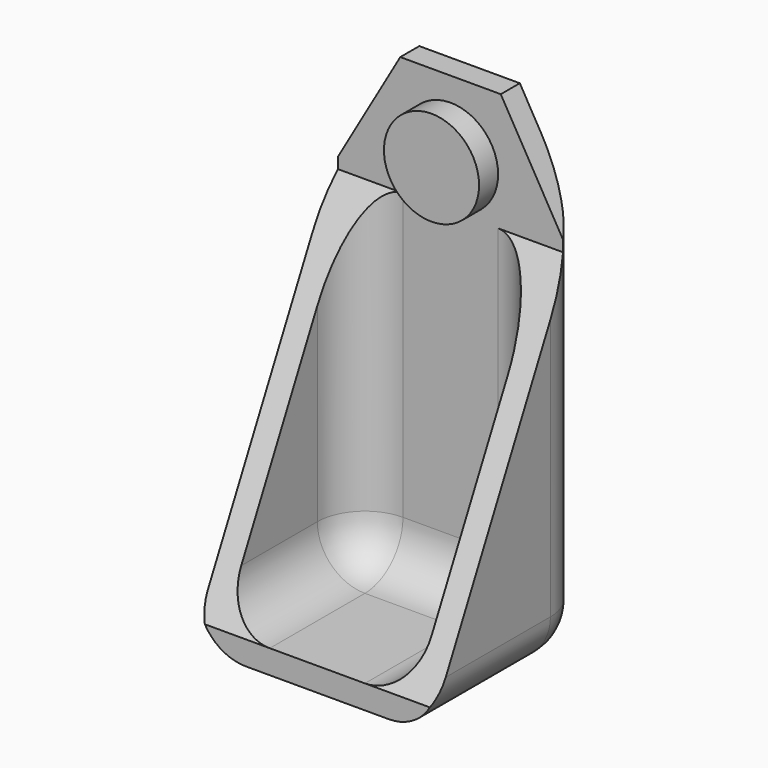
from build123d import *

# Parameters (mm, degrees)
F0_W          = 10
F0_H          = 15
F1_DEPTH      = 8
F2_W          = 8
F2_H          = 14
F3_DEPTH      = 14
F5_DEPTH      = 25
F7_DEPTH      = 1
F8_R          = 2
F9_DEPTH      = 1
F10_T1_DEPTH  = 4
F10_S5_W      = 2.04
F10_S5_H      = 2.04
F10_T6_DEPTH  = 2.04
F10_S11_W     = 2.04
F10_S11_H     = 2.04
F10_T12_DEPTH = 2.04
F10_T18_DEPTH = 10
F10_T23_DEPTH = 10
F10_T28_DEPTH = 17
F10_T33_DEPTH = 17
F10_T35_DEPTH = 6
F10_T37_DEPTH = 18
F10_T39_DEPTH = 11
F10_S43_W     = 2.04
F10_S43_H     = 2.04
F10_T44_DEPTH = 2.04
F10_S49_W     = 2.04
F10_S49_H     = 2.04
F10_T50_DEPTH = 2.04


# Not quite as in the source:
# - a fillet or chamfer that OpenCascade refuses, or shapes differently, is made with other operations: its cross-section is extruded or revolved along the edge and cut away or added


with BuildPart() as f1:
    # F0 (on Front) → F1 (new body)
    with BuildSketch(Plane.XZ):
        with Locations((0, 7.5)):
            Rectangle(F0_W, F0_H)
    extrude(amount=F1_DEPTH)

    # F2 (on face) → F3 (cut)
    with BuildSketch(Plane.XZ.offset(8)):
        with Locations((0, 8)):
            Rectangle(F2_W, F2_H)
    extrude(amount=-F3_DEPTH, mode=Mode.SUBTRACT)

    # F4 (on face) → F5 (cut)
    with BuildSketch(Plane(origin=(-5, 0, 0), x_dir=(0, -1, 0), z_dir=(-1, 0, 0))):
        Polygon((8, 15), (1, 15), (8, 1), align=None)
    extrude(amount=-F5_DEPTH, mode=Mode.SUBTRACT)

    # F6 (on face) → F7 (join)
    with BuildSketch(Plane(origin=(0, 0, 0), x_dir=(-1, 0, 0), z_dir=(0, 1, 0))):
        Polygon((4, 15), (5, 15), (2.1132486541, 20), (-2.1132486541, 20), (-5, 15), (-4, 15), (-4, 1), (4, 1), align=None)
    extrude(amount=-F7_DEPTH)

    # F8 (on face) → F9 (join)
    with BuildSketch(Plane.XZ.offset(1)):
        with Locations((0, 17)):
            Circle(F8_R)
    extrude(amount=F9_DEPTH)

    # F10: fillet of radius 2 on 12 edges, made by hand

    # F10_s2 → F10_t1 (join)
    with BuildSketch(Plane.YZ.offset(-2)):
        with BuildLine():
            ThreePointArc((-3, 1), (-1.5857864376, 1.5857864376), (-1, 3))
            Line((-1, 3), (-1, 1))
            Line((-1, 1), (-3, 1))
        make_face()
    extrude(amount=F10_T1_DEPTH)


with BuildPart() as f10_tool4:
    # F10_s5 → F10_t6 (new body)
    with BuildSketch(Plane.XY.offset(3)):
        with Locations((-3.02, -1.98)):
            Rectangle(F10_S5_W, F10_S5_H)
    extrude(amount=-F10_T6_DEPTH)

    # F10_s7 → F10_t8 (revolve, cut)
    with BuildSketch(Plane(origin=(-2, -3, 3), x_dir=(0.7071067812, -0.7071067812, 0), z_dir=(0.7071067812, 0.7071067812, 0))):
        with BuildLine():
            ThreePointArc((0, -2), (2, 0), (0, 2))
            Line((0, 2), (0, -2))
        make_face()
    revolve(axis=Axis((-2, -3, 3), (0, 0, -1)), mode=Mode.SUBTRACT)


with BuildPart() as f1_1:
    add(f1.part)

    # F10_t3: union F10_tool4
    add(f10_tool4.part)


with BuildPart() as f10_tool10:
    # F10_s11 → F10_t12 (new body)
    with BuildSketch(Plane.XY.offset(3)):
        with Locations((3.02, -1.98)):
            Rectangle(F10_S11_W, F10_S11_H)
    extrude(amount=-F10_T12_DEPTH)

    # F10_s13 → F10_t14 (revolve, cut)
    with BuildSketch(Plane(origin=(2, -3, 3), x_dir=(-0.7071067812, -0.7071067812, 0), z_dir=(0.7071067812, -0.7071067812, 0))):
        with BuildLine():
            ThreePointArc((0, -2), (2, 0), (0, 2))
            Line((0, 2), (0, -2))
        make_face()
    revolve(axis=Axis((2, -3, 3), (0, 0, -1)), mode=Mode.SUBTRACT)


with BuildPart() as f1_2:
    add(f1_1.part)

    # F10_t9: union F10_tool10
    add(f10_tool10.part)


with BuildPart() as f10_tool16:
    # F10_s17 → F10_t18 (new body)
    with BuildSketch(Plane.XZ.offset(13)):
        with BuildLine():
            ThreePointArc((-2, 1), (-3.4142135624, 1.5857864376), (-4, 3))
            Line((-4, 3), (-4, 1))
            Line((-4, 1), (-2, 1))
        make_face()
    extrude(amount=-F10_T18_DEPTH)

    split(bisect_by=Plane(origin=(0, -6.8, 3.4), x_dir=(1, 0, 0), z_dir=(0, 0.894427191, -0.4472135955)), keep=Keep.TOP)


with BuildPart() as f1_3:
    add(f1_2.part)

    # F10_t15: union F10_tool16
    add(f10_tool16.part)


with BuildPart() as f10_tool21:
    # F10_s22 → F10_t23 (new body)
    with BuildSketch(Plane.XZ.offset(13)):
        with BuildLine():
            ThreePointArc((2, 1), (3.4142135624, 1.5857864376), (4, 3))
            Line((4, 3), (4, 1))
            Line((4, 1), (2, 1))
        make_face()
    extrude(amount=-F10_T23_DEPTH)

    split(bisect_by=Plane(origin=(0, -6.8, 3.4), x_dir=(1, 0, 0), z_dir=(0, 0.894427191, -0.4472135955)), keep=Keep.TOP)


with BuildPart() as f1_4:
    add(f1_3.part)

    # F10_t20: union F10_tool21
    add(f10_tool21.part)


with BuildPart() as f10_tool26:
    # F10_s27 → F10_t28 (new body)
    with BuildSketch(Plane.XY.offset(20)):
        with BuildLine():
            ThreePointArc((2, -1), (3.4142135624, -1.5857864376), (4, -3))
            Line((4, -3), (4, -1))
            Line((4, -1), (2, -1))
        make_face()
    extrude(amount=-F10_T28_DEPTH)

    split(bisect_by=Plane(origin=(0, -6.8, 3.4), x_dir=(1, 0, 0), z_dir=(0, 0.894427191, -0.4472135955)), keep=Keep.TOP)


with BuildPart() as f1_5:
    add(f1_4.part)

    # F10_t25: union F10_tool26
    add(f10_tool26.part)


with BuildPart() as f10_tool31:
    # F10_s32 → F10_t33 (new body)
    with BuildSketch(Plane.XY.offset(3)):
        with BuildLine():
            ThreePointArc((-4, -3), (-3.4142135624, -1.5857864376), (-2, -1))
            Line((-2, -1), (-4, -1))
            Line((-4, -1), (-4, -3))
        make_face()
    extrude(amount=F10_T33_DEPTH)

    split(bisect_by=Plane(origin=(0, -6.8, 3.4), x_dir=(1, 0, 0), z_dir=(0, 0.894427191, -0.4472135955)), keep=Keep.TOP)


with BuildPart() as f1_6:
    add(f1_5.part)

    # F10_t30: union F10_tool31
    add(f10_tool31.part)

    # F10_s36 → F10_t35 (cut)
    with BuildSketch(Plane.YZ.offset(-3)):
        with BuildLine():
            ThreePointArc((-2, 0), (-0.5857864376, 0.5857864376), (0, 2))
            Line((0, 2), (0, 0))
            Line((0, 0), (-2, 0))
        make_face()
    extrude(amount=F10_T35_DEPTH, mode=Mode.SUBTRACT)

    # F10_s38 → F10_t37 (cut)
    with BuildSketch(Plane.XY.offset(2)):
        with BuildLine():
            ThreePointArc((-5, -2), (-4.4142135624, -0.5857864376), (-3, 0))
            Line((-3, 0), (-5, 0))
            Line((-5, 0), (-5, -2))
        make_face()
        with BuildLine():
            ThreePointArc((5, -2), (4.4142135624, -0.5857864376), (3, 0))
            Line((3, 0), (5, 0))
            Line((5, 0), (5, -2))
        make_face()
    extrude(amount=F10_T37_DEPTH, mode=Mode.SUBTRACT)

    # F10_s40 → F10_t39 (cut)
    with BuildSketch(Plane.XZ.offset(2)):
        with BuildLine():
            ThreePointArc((-5, 2), (-4.4142135624, 0.5857864376), (-3, 0))
            Line((-3, 0), (-5, 0))
            Line((-5, 0), (-5, 2))
        make_face()
        with BuildLine():
            ThreePointArc((5, 2), (4.4142135624, 0.5857864376), (3, 0))
            Line((3, 0), (5, 0))
            Line((5, 0), (5, 2))
        make_face()
    extrude(amount=F10_T39_DEPTH, mode=Mode.SUBTRACT)


with BuildPart() as f10_tool42:
    # F10_s43 → F10_t44 (new body)
    with BuildSketch(Plane.YZ.offset(-3)):
        with Locations((-0.98, 0.98)):
            Rectangle(F10_S43_W, F10_S43_H)
    extrude(amount=-F10_T44_DEPTH)

    # F10_s45 → F10_t46 (revolve, cut)
    with BuildSketch(Plane(origin=(-3, -2, 2), x_dir=(0, -0.7071067812, 0.7071067812), z_dir=(0, -0.7071067812, -0.7071067812))):
        with BuildLine():
            ThreePointArc((0, -2), (2, 0), (0, 2))
            Line((0, 2), (0, -2))
        make_face()
    revolve(axis=Axis((-3, -2, 2), (-1, 0, 0)), mode=Mode.SUBTRACT)


with BuildPart() as f1_7:
    add(f1_6.part)

    # F10_t41: cut F10_tool42
    add(f10_tool42.part, mode=Mode.SUBTRACT)


with BuildPart() as f10_tool48:
    # F10_s49 → F10_t50 (new body)
    with BuildSketch(Plane.YZ.offset(3)):
        with Locations((-0.98, 0.98)):
            Rectangle(F10_S49_W, F10_S49_H)
    extrude(amount=F10_T50_DEPTH)

    # F10_s51 → F10_t52 (revolve, cut)
    with BuildSketch(Plane(origin=(3, -2, 2), x_dir=(0, -0.7071067812, 0.7071067812), z_dir=(0, 0.7071067812, 0.7071067812))):
        with BuildLine():
            ThreePointArc((0, -2), (2, 0), (0, 2))
            Line((0, 2), (0, -2))
        make_face()
    revolve(axis=Axis((3, -2, 2), (1, 0, 0)), mode=Mode.SUBTRACT)


with BuildPart() as f1_8:
    add(f1_7.part)

    # F10_t47: cut F10_tool48
    add(f10_tool48.part, mode=Mode.SUBTRACT)


solid = f1_8.part
